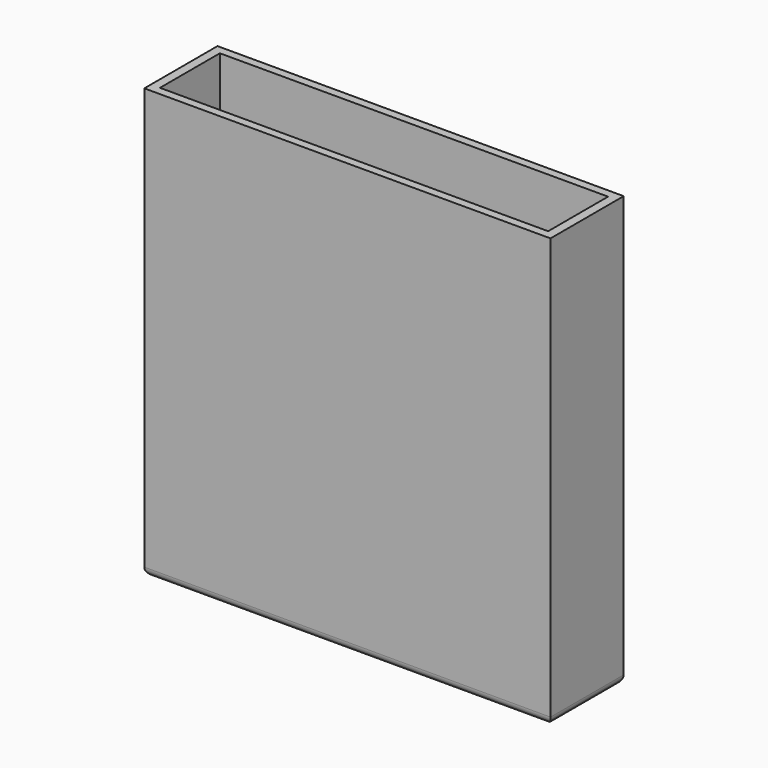
from build123d import *

# Parameters (mm, degrees)
F0_W     = 37.211
F0_H     = 39.37
F1_DEPTH = 4.191
F2_W     = 35.56
F2_H     = 6.858
F3_DEPTH = 39.37
F4_R     = 0.76199


# Not quite as in the source:
# - a fillet or chamfer is up to 0.001 mm smaller than in the source, because OpenCascade refuses the exact size


with BuildPart() as f1:
    # F0 (on Front) → F1 (new body, symmetric)
    with BuildSketch(Plane.XZ):
        Rectangle(F0_W, F0_H)
    extrude(amount=F1_DEPTH, both=True)

    # F2 (on face) → F3 (cut)
    with BuildSketch(Plane.XY.offset(19.685)):
        Rectangle(F2_W, F2_H)
    extrude(amount=-F3_DEPTH, mode=Mode.SUBTRACT)

    # F4 (radius 0.762 in the source; OpenCascade refuses exactly that, so slightly less here)
    f4_edges = [f1.edges().sort_by_distance(p)[0] for p in [
        (0, -4.191, -19.685),
        (18.6055, 0, -19.685),
        (0, 4.191, -19.685),
        (-18.6055, 0, -19.685),
    ]]
    fillet(f4_edges, radius=F4_R)


solid = f1.part
